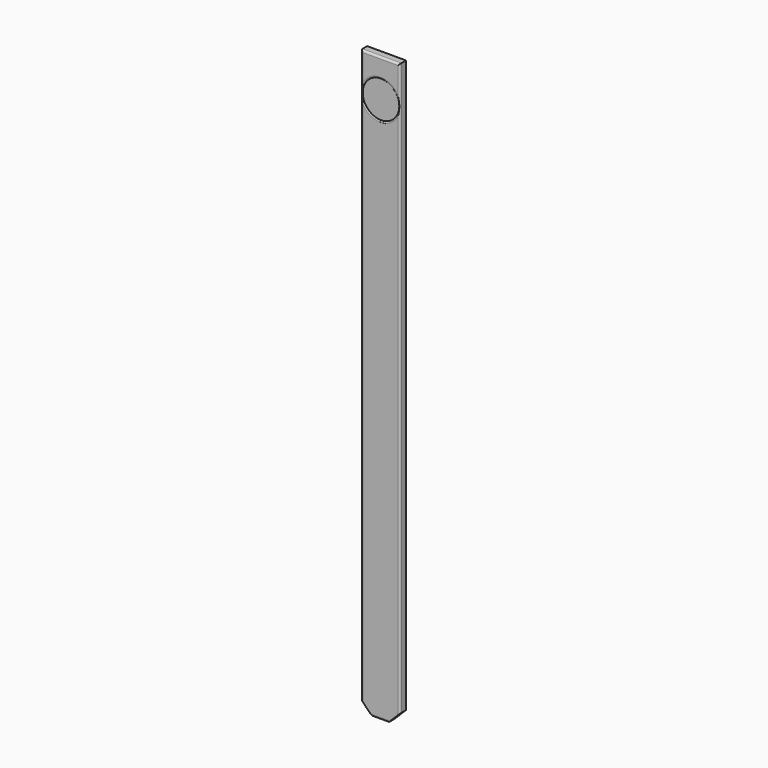
from build123d import *

# Parameters (mm, degrees)
F0_W        = 100
F0_H        = 20
F1_DEPTH    = 750
F2_R        = 47
F3_DEPTH    = 2
F4_W        = 70
F4_H        = 1470
F5_DEPTH    = 15
F6_T1_DEPTH = 70
F6_T3_DEPTH = 1470
F7_T1_DEPTH = 125
F7_T3_DEPTH = 1525
F8_T1_DEPTH = 169.300979278


# Not quite as in the source:
# - a fillet or chamfer that OpenCascade refuses, or shapes differently, is made with other operations: its cross-section is extruded or revolved along the edge and cut away or added


with BuildPart() as f1:
    # F0 (on Top) → F1 (new body, symmetric)
    with BuildSketch(Plane.XY):
        Rectangle(F0_W, F0_H)
    extrude(amount=F1_DEPTH, both=True)

    # F2 (on face) → F3 (cut)
    with BuildSketch(Plane.XZ.offset(10)):
        with Locations((0, 653)):
            Circle(F2_R)
    extrude(amount=-F3_DEPTH, mode=Mode.SUBTRACT)

    # F4 (on face) → F5 (cut)
    with BuildSketch(Plane(origin=(0, 10, 0), x_dir=(-1, 0, 0), z_dir=(0, 1, 0))):
        Rectangle(F4_W, F4_H)
    extrude(amount=-F5_DEPTH, mode=Mode.SUBTRACT)

    # F6: fillet of radius 30 on 4 edges, made by hand

    # F6_s2 → F6_t1 (join)
    with BuildSketch(Plane.YZ.offset(-35)):
        with BuildLine():
            ThreePointArc((10, 735), (-0.9807621135, 724.0192378865), (-5, 709.0192378865))
            Line((-5, 709.0192378865), (-5, 735))
            Line((-5, 735), (10, 735))
        make_face()
        with BuildLine():
            ThreePointArc((10, -735), (-0.9807621135, -724.0192378865), (-5, -709.0192378865))
            Line((-5, -709.0192378865), (-5, -735))
            Line((-5, -735), (10, -735))
        make_face()
    extrude(amount=F6_T1_DEPTH)

    # F6_s4 → F6_t3 (join)
    with BuildSketch(Plane.XY.offset(-735)):
        with BuildLine():
            ThreePointArc((35, 10), (24.0192378865, -0.9807621135), (9.0192378865, -5))
            Line((9.0192378865, -5), (35, -5))
            Line((35, -5), (35, 10))
        make_face()
        with BuildLine():
            ThreePointArc((-35, 10), (-24.0192378865, -0.9807621135), (-9.0192378865, -5))
            Line((-9.0192378865, -5), (-35, -5))
            Line((-35, -5), (-35, 10))
        make_face()
    extrude(amount=F6_T3_DEPTH)

    # F7: fillet of radius 5 on 5 edges, made by hand

    # F7_s2 → F7_t1 (cut)
    with BuildSketch(Plane.YZ.offset(-62.5)):
        with BuildLine():
            ThreePointArc((-10, -745), (-8.5355339059, -748.5355339059), (-5, -750))
            Line((-5, -750), (-10, -750))
            Line((-10, -750), (-10, -745))
        make_face()
        with BuildLine():
            ThreePointArc((-10, 745), (-8.5355339059, 748.5355339059), (-5, 750))
            Line((-5, 750), (-10, 750))
            Line((-10, 750), (-10, 745))
        make_face()
    extrude(amount=F7_T1_DEPTH, mode=Mode.SUBTRACT)

    # F7_s4 → F7_t3 (cut)
    with BuildSketch(Plane.XY.offset(-762.5)):
        with BuildLine():
            ThreePointArc((-45, -10), (-48.5355339059, -8.5355339059), (-50, -5))
            Line((-50, -5), (-50, -10))
            Line((-50, -10), (-45, -10))
        make_face()
        with BuildLine():
            ThreePointArc((45, -10), (48.5355339059, -8.5355339059), (50, -5))
            Line((50, -5), (50, -10))
            Line((50, -10), (45, -10))
        make_face()
    extrude(amount=F7_T3_DEPTH, mode=Mode.SUBTRACT)

    # F7_s5 → F7_t6 (revolve, cut)
    with BuildSketch(Plane.XY.offset(653)):
        with BuildLine():
            ThreePointArc((51, -10), (48.7639320225, -9.472135955), (47, -8))
            Line((47, -8), (47, -10))
            Line((47, -10), (51, -10))
        make_face()
    revolve(axis=Axis((0, -10, 653), (0, -1, 0)), mode=Mode.SUBTRACT)

    # F8: chamfer of 30 on 2 edges, made by hand

    # F8_s2 → F8_t1 (cut)
    with BuildSketch(Plane.XZ.offset(-87.150489639)):
        Polygon((50, -720), (20, -750), (50, -750), align=None)
        Polygon((-50, -720), (-20, -750), (-50, -750), align=None)
    extrude(amount=F8_T1_DEPTH, mode=Mode.SUBTRACT)


solid = f1.part
